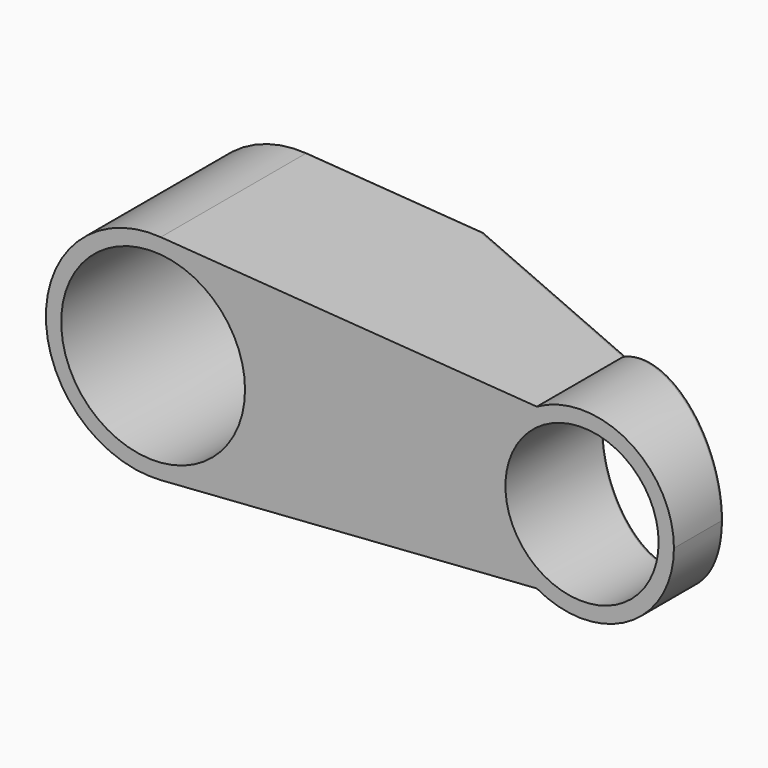
from build123d import *

# Parameters (mm, degrees)
F0_R     = 30
F1_DEPTH = 60
F3_DEPTH = 45
F4_R     = 0.99999


# Not quite as in the source:
# - a fillet or chamfer is up to 0.001 mm smaller than in the source, because OpenCascade refuses the exact size


with BuildPart() as f1:
    # F0 (on Front) → F1 (new body)
    with BuildSketch(Plane.XZ):
        with BuildLine():
            ThreePointArc((2.5, -34.9106001094), (25.6173769149, -23.8484800354), (35, 0))
            ThreePointArc((35, 0), (25.6173769149, 23.8484800354), (2.5, 34.9106001094))
            ThreePointArc((2.5, 34.9106001094), (-35, 0), (2.5, -34.9106001094))
        make_face()
        Circle(F0_R, mode=Mode.SUBTRACT)
        with BuildLine():
            ThreePointArc((2.5, 34.9106001094), (25.6173769149, 23.8484800354), (35, 0))
            ThreePointArc((35, 0), (25.6173769149, -23.8484800354), (2.5, -34.9106001094))
            Line((2.5, -34.9106001094), (125.2449483187, -26.120651789))
            ThreePointArc((125.2449483187, -26.120651789), (110, 0), (125.2449483187, 26.120651789))
            Line((125.2449483187, 26.120651789), (2.5, 34.9106001094))
        make_face()
        with BuildLine():
            ThreePointArc((170, 0), (155.1219782033, 25.9099551374), (125.2449483187, 26.120651789))
            Line((125.2449483187, 26.120651789), (141.7857142857, 24.9361429353))
            ThreePointArc((141.7857142857, 24.9361429353), (158.2981263678, 17.0346285967), (165, 0))
            ThreePointArc((165, 0), (158.2981263678, -17.0346285967), (141.7857142857, -24.9361429353))
            Line((141.7857142857, -24.9361429353), (125.2449483187, -26.120651789))
            ThreePointArc((125.2449483187, -26.120651789), (155.1219782033, -25.9099551373), (170, 0))
        make_face()
        with BuildLine():
            Line((141.7857142857, 24.9361429353), (125.2449483187, 26.120651789))
            ThreePointArc((125.2449483187, 26.120651789), (110, 0), (125.2449483187, -26.120651789))
            Line((125.2449483187, -26.120651789), (141.7857142857, -24.9361429353))
            ThreePointArc((141.7857142857, -24.9361429353), (115, 0), (141.7857142857, 24.9361429353))
        make_face()
    extrude(amount=F1_DEPTH)

    # F2 (on Top) → F3 (cut, symmetric)
    with BuildSketch(Plane.XY):
        Polygon((194.0050084083, -48.808039949), (194.0050084083, 0), (59.9060207605, 0), align=None)
    extrude(amount=F3_DEPTH, both=True, mode=Mode.SUBTRACT)

    # F4 (radius 1 in the source; OpenCascade refuses exactly that, so slightly less here)
    f4_edges = [f1.edges().sort_by_distance(p)[0] for p in [
        (138.214248, -28.501864, -24.93614),
        (92.575485, -11.890712, 28.460161),
        (170, -40.070931, 1e-06),
        (92.575485, -11.890712, -28.460161),
        (-30, 0, 0),
        (31.20301, 0, 32.855135),
        (-35, 0, 0),
        (31.20301, 0, -32.855135),
    ]]
    fillet(f4_edges, radius=F4_R)


solid = f1.part
